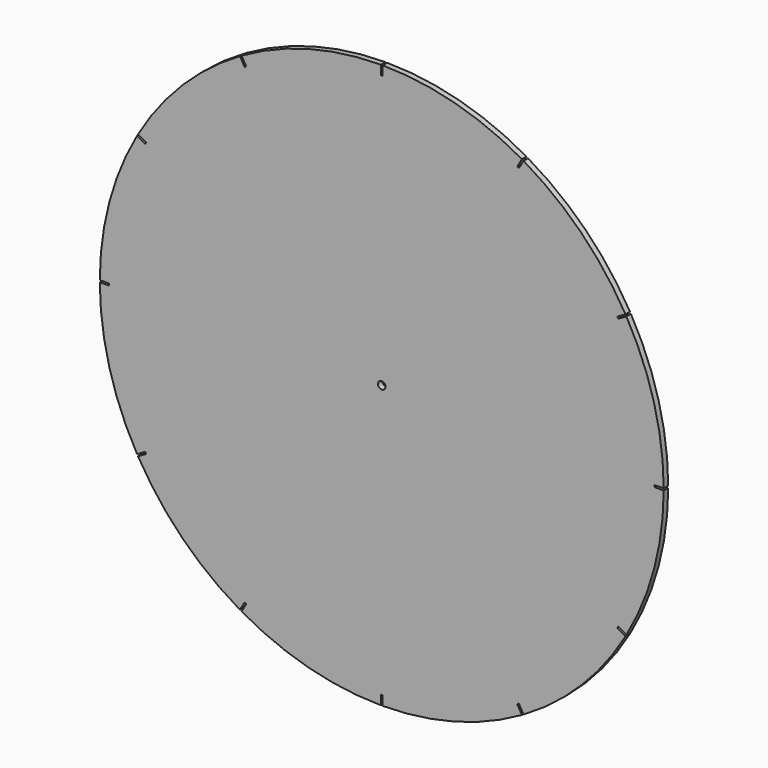
from build123d import *

# Parameters (mm, degrees)
F0_R            = 150
F0_R_2          = 2
F1_DEPTH        = 3
F2_W            = 1
F2_H            = 6.1217802763
F3_DEPTH        = 18.2
F3_COPIES_COUNT = 12


# Not quite as in the source:
# - a pattern or mirror of a feature is missing from the dataset's text; its kind, count and spacing are read off the source's solid


with BuildPart() as f1:
    # F0 (on Front) → F1 (new body)
    with BuildSketch(Plane.XZ):
        Circle(F0_R)
        Circle(F0_R_2, mode=Mode.SUBTRACT)
    extrude(amount=F1_DEPTH)

    # F2 (on Front) → F3 (cut)
    with BuildSketch(Plane.XZ):
        with Locations((0, 148.0608901381)):
            Rectangle(F2_W, F2_H)
    f3 = extrude(amount=F3_DEPTH, mode=Mode.SUBTRACT)

    # F3_copies: F3 ×12 about axis
    f3_copies_axis = Axis((0, 0, 0), (0, 1, 0))
    for i in range(1, F3_COPIES_COUNT):
        add(f3.rotate(f3_copies_axis, i * 360 / F3_COPIES_COUNT), mode=Mode.SUBTRACT)


solid = f1.part
